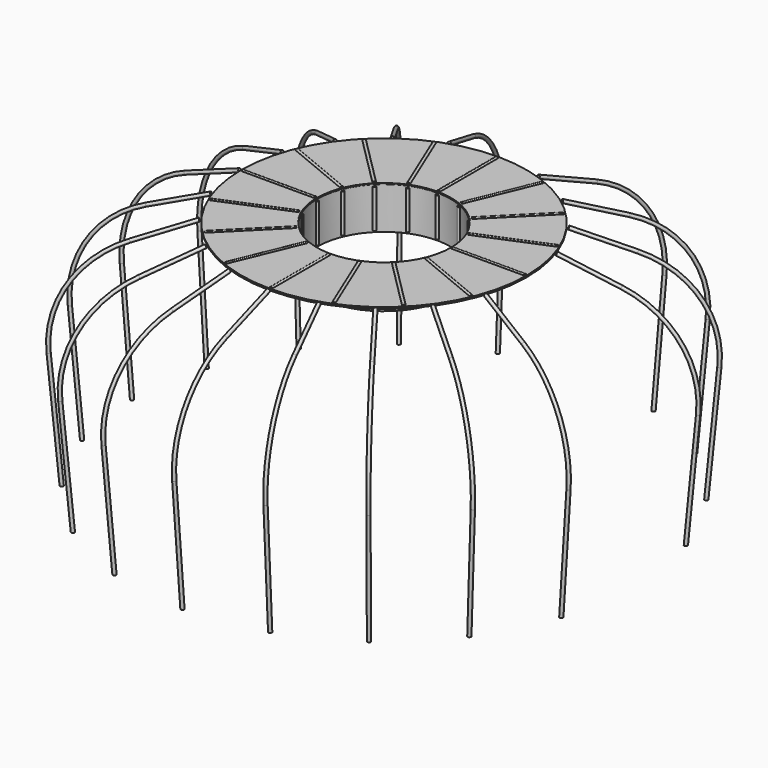
from build123d import *

# Parameters (mm, degrees)
F4_R      = 10
F5_DEPTH  = 430
F7_R      = 10
F8_DEPTH  = 230
F9_COUNT  = 16
F11_R     = 10
F13_COUNT = 20
F14_W     = 3326.876282692
F14_H     = 1645.6206440926
F15_DEPTH = 2000
F16_R     = 850
F16_R_2   = 400
F17_DEPTH = 5
F18_W     = 5
F18_H     = 250


# Not quite as in the source:
# - an extrude ends at something that could not be found from the text; its depth is read off the source's solid
# - the program builds the solid bodies; features that only make, move or delete a surface that nothing else refers to are left out


with BuildPart() as f5:
    # F4 (on plane+point) → F5 (new body, through all)
    with BuildSketch(Plane.YZ.offset(-410)):
        with Locations((0, 1410)):
            Circle(F4_R)
    extrude(amount=-F5_DEPTH)


with BuildPart() as f8:
    # F7 (on plane+point) → F8 (new body, through all)
    with BuildSketch(Plane.XY.offset(1170)):
        with Locations((-400, 0)):
            Circle(F7_R)
    extrude(amount=F8_DEPTH)


with BuildPart() as f9_1:
    # F9: instance of F8
    add(f8.part.rotate(Axis((0, 0, 700), (0, 0, 1)), 1 * 360 / F9_COUNT))


with BuildPart() as f9_2:
    # F9: instance of F8
    add(f8.part.rotate(Axis((0, 0, 700), (0, 0, 1)), 2 * 360 / F9_COUNT))


with BuildPart() as f9_3:
    # F9: instance of F8
    add(f8.part.rotate(Axis((0, 0, 700), (0, 0, 1)), 3 * 360 / F9_COUNT))


with BuildPart() as f9_4:
    # F9: instance of F8
    add(f8.part.rotate(Axis((0, 0, 700), (0, 0, 1)), 4 * 360 / F9_COUNT))


with BuildPart() as f9_5:
    # F9: instance of F8
    add(f8.part.rotate(Axis((0, 0, 700), (0, 0, 1)), 5 * 360 / F9_COUNT))


with BuildPart() as f9_6:
    # F9: instance of F8
    add(f8.part.rotate(Axis((0, 0, 700), (0, 0, 1)), 6 * 360 / F9_COUNT))


with BuildPart() as f9_7:
    # F9: instance of F8
    add(f8.part.rotate(Axis((0, 0, 700), (0, 0, 1)), 7 * 360 / F9_COUNT))


with BuildPart() as f9_8:
    # F9: instance of F8
    add(f8.part.rotate(Axis((0, 0, 700), (0, 0, 1)), 8 * 360 / F9_COUNT))


with BuildPart() as f9_9:
    # F9: instance of F8
    add(f8.part.rotate(Axis((0, 0, 700), (0, 0, 1)), 9 * 360 / F9_COUNT))


with BuildPart() as f9_10:
    # F9: instance of F8
    add(f8.part.rotate(Axis((0, 0, 700), (0, 0, 1)), 10 * 360 / F9_COUNT))


with BuildPart() as f9_11:
    # F9: instance of F8
    add(f8.part.rotate(Axis((0, 0, 700), (0, 0, 1)), 11 * 360 / F9_COUNT))


with BuildPart() as f9_12:
    # F9: instance of F8
    add(f8.part.rotate(Axis((0, 0, 700), (0, 0, 1)), 12 * 360 / F9_COUNT))


with BuildPart() as f9_13:
    # F9: instance of F8
    add(f8.part.rotate(Axis((0, 0, 700), (0, 0, 1)), 13 * 360 / F9_COUNT))


with BuildPart() as f9_14:
    # F9: instance of F8
    add(f8.part.rotate(Axis((0, 0, 700), (0, 0, 1)), 14 * 360 / F9_COUNT))


with BuildPart() as f9_15:
    # F9: instance of F8
    add(f8.part.rotate(Axis((0, 0, 700), (0, 0, 1)), 15 * 360 / F9_COUNT))


with BuildPart() as f9_16:
    # F9: instance of F5
    add(f5.part.rotate(Axis((0, 0, 700), (0, 0, 1)), 1 * 360 / F9_COUNT))


with BuildPart() as f9_17:
    # F9: instance of F5
    add(f5.part.rotate(Axis((0, 0, 700), (0, 0, 1)), 2 * 360 / F9_COUNT))


with BuildPart() as f9_18:
    # F9: instance of F5
    add(f5.part.rotate(Axis((0, 0, 700), (0, 0, 1)), 3 * 360 / F9_COUNT))


with BuildPart() as f9_19:
    # F9: instance of F5
    add(f5.part.rotate(Axis((0, 0, 700), (0, 0, 1)), 4 * 360 / F9_COUNT))


with BuildPart() as f9_20:
    # F9: instance of F5
    add(f5.part.rotate(Axis((0, 0, 700), (0, 0, 1)), 5 * 360 / F9_COUNT))


with BuildPart() as f9_21:
    # F9: instance of F5
    add(f5.part.rotate(Axis((0, 0, 700), (0, 0, 1)), 6 * 360 / F9_COUNT))


with BuildPart() as f9_22:
    # F9: instance of F5
    add(f5.part.rotate(Axis((0, 0, 700), (0, 0, 1)), 7 * 360 / F9_COUNT))


with BuildPart() as f9_23:
    # F9: instance of F5
    add(f5.part.rotate(Axis((0, 0, 700), (0, 0, 1)), 8 * 360 / F9_COUNT))


with BuildPart() as f9_24:
    # F9: instance of F5
    add(f5.part.rotate(Axis((0, 0, 700), (0, 0, 1)), 9 * 360 / F9_COUNT))


with BuildPart() as f9_25:
    # F9: instance of F5
    add(f5.part.rotate(Axis((0, 0, 700), (0, 0, 1)), 10 * 360 / F9_COUNT))


with BuildPart() as f9_26:
    # F9: instance of F5
    add(f5.part.rotate(Axis((0, 0, 700), (0, 0, 1)), 11 * 360 / F9_COUNT))


with BuildPart() as f9_27:
    # F9: instance of F5
    add(f5.part.rotate(Axis((0, 0, 700), (0, 0, 1)), 12 * 360 / F9_COUNT))


with BuildPart() as f9_28:
    # F9: instance of F5
    add(f5.part.rotate(Axis((0, 0, 700), (0, 0, 1)), 13 * 360 / F9_COUNT))


with BuildPart() as f9_29:
    # F9: instance of F5
    add(f5.part.rotate(Axis((0, 0, 700), (0, 0, 1)), 14 * 360 / F9_COUNT))


with BuildPart() as f9_30:
    # F9: instance of F5
    add(f5.part.rotate(Axis((0, 0, 700), (0, 0, 1)), 15 * 360 / F9_COUNT))


with BuildPart() as f12:
    # F12: sweep along a path in F0
    with BuildLine(Plane.XZ) as f12_path:
        Line((-1500, 0), (-1561.0090199234, 697.3362886642))
        ThreePointArc((-1561.0090199234, 697.3362886642), (-1472.3747487227, 1059.5546584708), (-1181.5518811848, 1292.9646864764))
        Line((-1181.5518811848, 1292.9646864764), (-860, 1410))
    # F11 (on offset) → F12 (sweep)
    with BuildSketch(Plane.XY.offset(10)):
        with Locations((-1500.8715574275, 0)):
            Circle(F11_R)
    sweep(path=f12_path.line)


with BuildPart() as f13_1:
    # F13: instance of F12
    add(f12.part.rotate(Axis((0, 0, 700), (0, 0, 1)), 1 * 360 / F13_COUNT))


with BuildPart() as f13_2:
    # F13: instance of F12
    add(f12.part.rotate(Axis((0, 0, 700), (0, 0, 1)), 2 * 360 / F13_COUNT))


with BuildPart() as f13_3:
    # F13: instance of F12
    add(f12.part.rotate(Axis((0, 0, 700), (0, 0, 1)), 3 * 360 / F13_COUNT))


with BuildPart() as f13_4:
    # F13: instance of F12
    add(f12.part.rotate(Axis((0, 0, 700), (0, 0, 1)), 4 * 360 / F13_COUNT))


with BuildPart() as f13_5:
    # F13: instance of F12
    add(f12.part.rotate(Axis((0, 0, 700), (0, 0, 1)), 5 * 360 / F13_COUNT))


with BuildPart() as f13_6:
    # F13: instance of F12
    add(f12.part.rotate(Axis((0, 0, 700), (0, 0, 1)), 6 * 360 / F13_COUNT))


with BuildPart() as f13_7:
    # F13: instance of F12
    add(f12.part.rotate(Axis((0, 0, 700), (0, 0, 1)), 7 * 360 / F13_COUNT))


with BuildPart() as f13_8:
    # F13: instance of F12
    add(f12.part.rotate(Axis((0, 0, 700), (0, 0, 1)), 8 * 360 / F13_COUNT))


with BuildPart() as f13_9:
    # F13: instance of F12
    add(f12.part.rotate(Axis((0, 0, 700), (0, 0, 1)), 9 * 360 / F13_COUNT))


with BuildPart() as f13_10:
    # F13: instance of F12
    add(f12.part.rotate(Axis((0, 0, 700), (0, 0, 1)), 10 * 360 / F13_COUNT))


with BuildPart() as f13_11:
    # F13: instance of F12
    add(f12.part.rotate(Axis((0, 0, 700), (0, 0, 1)), 11 * 360 / F13_COUNT))


with BuildPart() as f13_12:
    # F13: instance of F12
    add(f12.part.rotate(Axis((0, 0, 700), (0, 0, 1)), 12 * 360 / F13_COUNT))


with BuildPart() as f13_13:
    # F13: instance of F12
    add(f12.part.rotate(Axis((0, 0, 700), (0, 0, 1)), 13 * 360 / F13_COUNT))


with BuildPart() as f13_14:
    # F13: instance of F12
    add(f12.part.rotate(Axis((0, 0, 700), (0, 0, 1)), 14 * 360 / F13_COUNT))


with BuildPart() as f13_15:
    # F13: instance of F12
    add(f12.part.rotate(Axis((0, 0, 700), (0, 0, 1)), 15 * 360 / F13_COUNT))


with BuildPart() as f13_16:
    # F13: instance of F12
    add(f12.part.rotate(Axis((0, 0, 700), (0, 0, 1)), 16 * 360 / F13_COUNT))


with BuildPart() as f13_17:
    # F13: instance of F12
    add(f12.part.rotate(Axis((0, 0, 700), (0, 0, 1)), 17 * 360 / F13_COUNT))


with BuildPart() as f13_18:
    # F13: instance of F12
    add(f12.part.rotate(Axis((0, 0, 700), (0, 0, 1)), 18 * 360 / F13_COUNT))


with BuildPart() as f13_19:
    # F13: instance of F12
    add(f12.part.rotate(Axis((0, 0, 700), (0, 0, 1)), 19 * 360 / F13_COUNT))


with BuildPart() as f15_tool:
    # F14 (on Front) → F15 (new body, symmetric)
    with BuildSketch(Plane.XZ):
        with Locations((33.4325432777, 686.81666255)):
            Rectangle(F14_W, F14_H)
    extrude(amount=F15_DEPTH, both=True)


with BuildPart() as f13_10_1:
    add(f13_10.part)

    # F15: cut by f15_tool
    add(f15_tool.part, mode=Mode.SUBTRACT)


with BuildPart() as f13_15_1:
    add(f13_15.part)

    # F15: cut by f15_tool
    add(f15_tool.part, mode=Mode.SUBTRACT)


with BuildPart() as f17:
    # F16 (on line) → F17 (new body, symmetric)
    with BuildSketch(Plane(origin=(0, 0, 1410), x_dir=(1, 0, 0), z_dir=(0, 0, -1))):
        Circle(F16_R)
        Circle(F16_R_2, mode=Mode.SUBTRACT)
    extrude(amount=F17_DEPTH, both=True)


with BuildPart() as f19:
    # F18 (on Front) → F19 (revolve)
    with BuildSketch(Plane.XZ):
        with Locations((-400, 1285)):
            Rectangle(F18_W, F18_H)
    revolve(axis=Axis((0, 0, 700), (0, 0, 1)))


solid = Compound([f5.part, f8.part, f9_1.part, f9_2.part, f9_3.part, f9_4.part, f9_5.part, f9_6.part, f9_7.part, f9_8.part, f9_9.part, f9_10.part, f9_11.part, f9_12.part, f9_13.part, f9_14.part, f9_15.part, f9_16.part, f9_17.part, f9_18.part, f9_19.part, f9_20.part, f9_21.part, f9_22.part, f9_23.part, f9_24.part, f9_25.part, f9_26.part, f9_27.part, f9_28.part, f9_29.part, f9_30.part, f12.part, f13_1.part, f13_2.part, f13_3.part, f13_4.part, f13_5.part, f13_6.part, f13_7.part, f13_8.part, f13_9.part, f13_11.part, f13_12.part, f13_13.part, f13_14.part, f13_16.part, f13_17.part, f13_18.part, f13_19.part, f17.part, f19.part])
